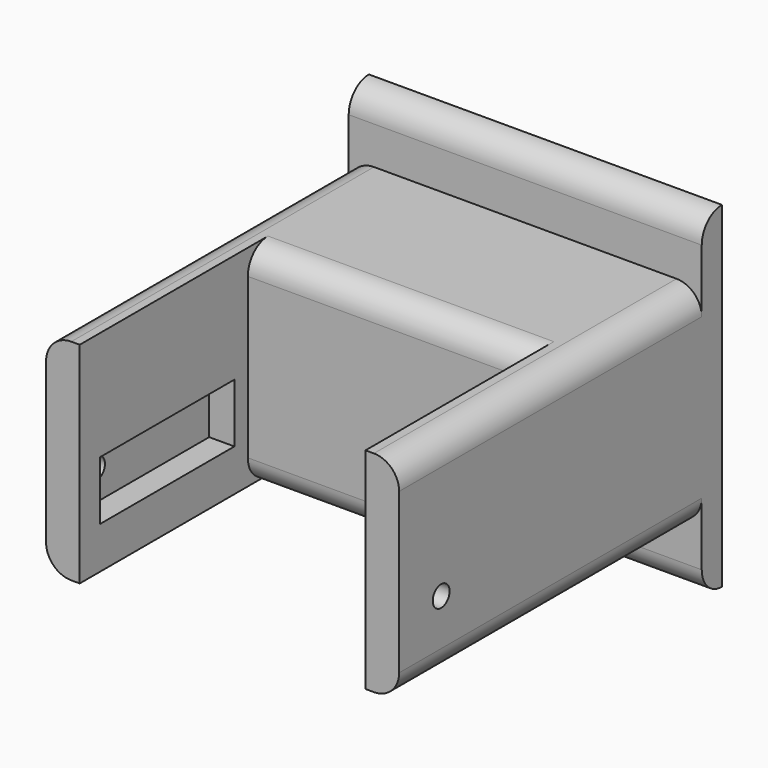
from build123d import *

# Parameters (mm, degrees)
F0_W     = 42
F0_H     = 40
F1_DEPTH = 3
F2_W     = 42
F2_H     = 25
F3_DEPTH = 45
F4_W     = 34
F4_H     = 25
F5_DEPTH = 32.501
F6_W     = 20
F6_H     = 7
F7_DEPTH = 3
F8_R     = 1.25
F9_DEPTH = 42.001
F10_R    = 2.99999


# Not quite as in the source:
# - a fillet or chamfer is up to 0.001 mm smaller than in the source, because OpenCascade refuses the exact size


with BuildPart() as f1:
    # F0 (on Front) → F1 (new body)
    with BuildSketch(Plane.XZ):
        with Locations((-2.4715067595, 12.8215752275)):
            Rectangle(F0_W, F0_H)
    extrude(amount=F1_DEPTH)

    # F2 (on face) → F3 (join)
    with BuildSketch(Plane.XZ.offset(3)):
        with Locations((-2.4715067595, 12.8215752275)):
            Rectangle(F2_W, F2_H)
    extrude(amount=F3_DEPTH)

    # F4 (on face) → F5 (cut, through all)
    with BuildSketch(Plane(origin=(0, 0, 0.3215752275), x_dir=(1, 0, 0), z_dir=(0, 0, -1))):
        with Locations((-2.4715067595, 35.5)):
            Rectangle(F4_W, F4_H)
    extrude(amount=-F5_DEPTH, mode=Mode.SUBTRACT)

    # F6 (on face) → F7 (cut)
    with BuildSketch(Plane.YZ.offset(-19.4715067595)):
        with Locations((-35, 8.8215752275)):
            Rectangle(F6_W, F6_H)
    extrude(amount=-F7_DEPTH, mode=Mode.SUBTRACT)

    # F8 (on face) → F9 (cut, through all)
    with BuildSketch(Plane(origin=(-23.4715067595, 0, 0), x_dir=(0, -1, 0), z_dir=(-1, 0, 0))):
        with Locations((41.75, 8.8215752275)):
            Circle(F8_R)
    extrude(amount=-F9_DEPTH, mode=Mode.SUBTRACT)

    # F10 (radius 3 in the source; OpenCascade refuses exactly that, so slightly less here)
    f10_edges = [f1.edges().sort_by_distance(p)[0] for p in [
        (-23.471507, -25.5, 0.321575),
        (18.528493, -25.5, 0.321575),
        (-23.471507, -25.5, 25.321575),
        (18.528493, -25.5, 25.321575),
        (-2.471507, -23, 25.321575),
        (-2.471507, -23, 0.321575),
        (-2.471507, -3, -7.178425),
        (-2.471507, -3, 32.821575),
    ]]
    fillet(f10_edges, radius=F10_R)


solid = f1.part
